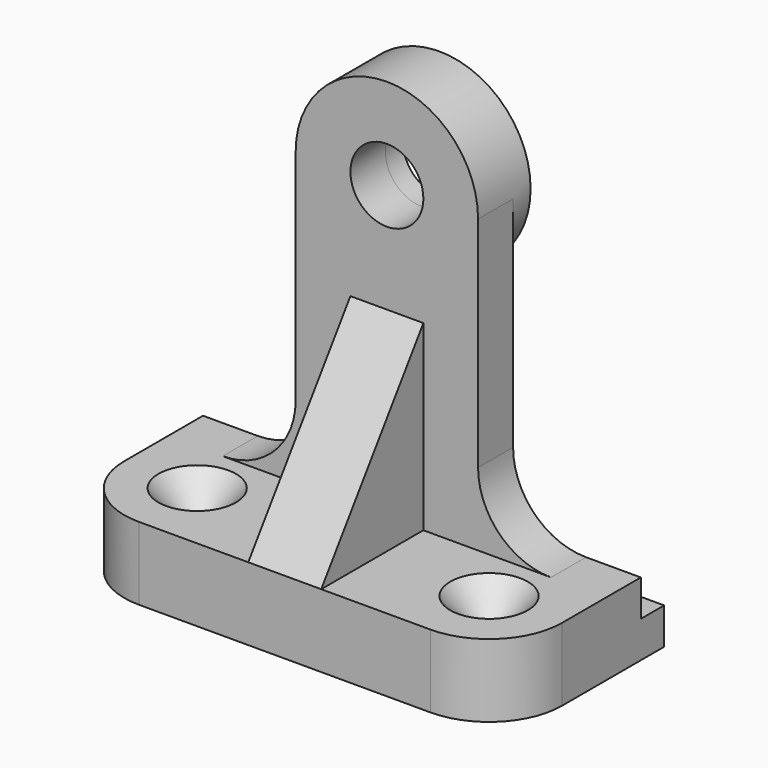
from build123d import *

# Parameters (mm, degrees)
F1_DEPTH        = 29.845
F0_R            = 6.35
F2_DEPTH        = 7.62
F3_W            = 76.2
F3_H            = 6.35
F4_DEPTH        = 5.08
F5_R            = 6.35
F6_DEPTH        = 3.81
F8_DEPTH        = 6.35
F9_R            = 12.7
F11_D           = 5.1054
F11_CSINK_D     = 13.4874
F11_CSINK_ANGLE = 82


with BuildPart() as f1:
    # F0 (on Front) → F1 (new body)
    with BuildSketch(Plane.XZ):
        Polygon((38.1, -50.8), (28.575, -50.8), (-28.575, -50.8), (-38.1, -50.8), (-38.1, -63.5), (38.1, -63.5), align=None)
    extrude(amount=F1_DEPTH)

    # F0 (on Front) → F2 (join)
    with BuildSketch(Plane.XZ):
        with BuildLine():
            Line((15.875, -38.1), (15.875, 0))
            ThreePointArc((15.875, 0), (0, 15.875), (-15.875, 0))
            Line((-15.875, 0), (-15.875, -38.1))
            ThreePointArc((-15.875, -38.1), (-19.5947438789, -47.0802561211), (-28.575, -50.8))
            Line((-28.575, -50.8), (28.575, -50.8))
            ThreePointArc((28.575, -50.8), (19.5947438789, -47.0802561211), (15.875, -38.1))
        make_face()
        Circle(F0_R, mode=Mode.SUBTRACT)
    extrude(amount=F2_DEPTH)

    # F3 (on face) → F4 (join)
    with BuildSketch(Plane(origin=(0, 0, 0), x_dir=(-1, 0, 0), z_dir=(0, 1, 0))):
        with Locations((0, -60.325)):
            Rectangle(F3_W, F3_H)
    extrude(amount=F4_DEPTH)

    # F5 (on face) → F6 (join)
    with BuildSketch(Plane(origin=(0, 0, 0), x_dir=(-1, 0, 0), z_dir=(0, 1, 0))):
        with BuildLine():
            ThreePointArc((15.875, 0), (0, 15.875), (-15.875, 0))
            ThreePointArc((-15.875, 0), (0, -15.875), (15.875, 0))
        make_face()
        Circle(F5_R, mode=Mode.SUBTRACT)
    extrude(amount=F6_DEPTH)

    # F7 (on Right) → F8 (join, symmetric)
    with BuildSketch(Plane.YZ):
        Polygon((-7.62, -50.8), (-7.62, -19.05), (-29.845, -50.8), align=None)
    extrude(amount=F8_DEPTH, both=True)

    # F9
    f9_edges = [f1.edges().sort_by_distance(p)[0] for p in [
        (-38.1, -29.845, -57.15),
        (38.1, -29.845, -57.15),
    ]]
    fillet(f9_edges, radius=F9_R)

    # F11 (through all)
    with Locations(Plane.XY.offset(-50.8)):
        with Locations((25.4, -17.145), (-25.4, -17.145)):
            CounterSinkHole(F11_D / 2, F11_CSINK_D / 2, counter_sink_angle=F11_CSINK_ANGLE)


solid = f1.part
